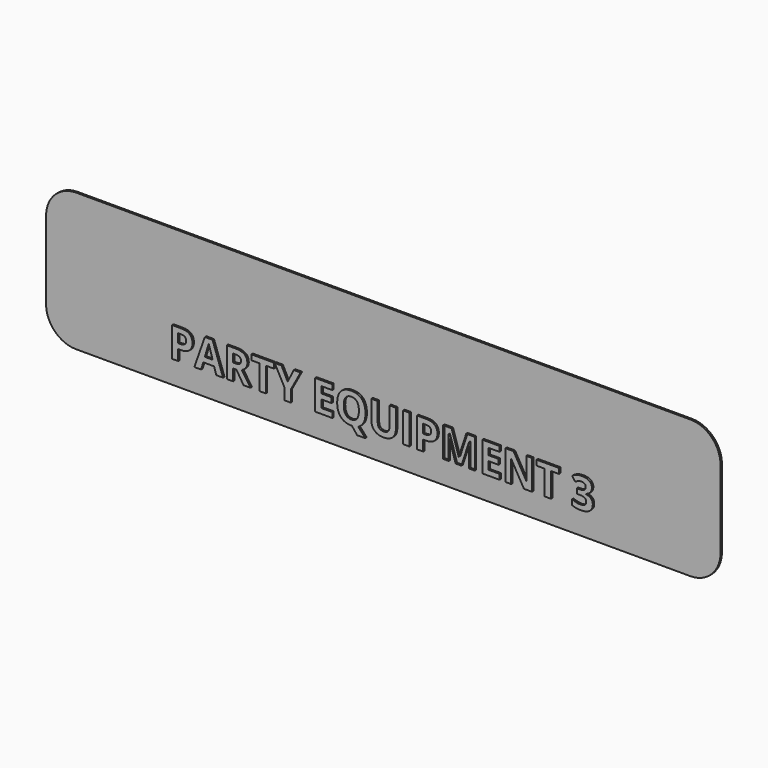
from build123d import *

# Parameters (mm, degrees)
F1_DEPTH     = 0.6
F2_TEXT_SIZE = 13.8888888889
F3_DEPTH     = 0.6


# Not quite as in the source:
# - Text() gives the source's letters only with a copy of the font that has no kerning and outlines rounded to 1/6400 em; it was checked with that copy


with BuildPart() as f1:
    # F0 (on Front) → F1 (new body)
    with BuildSketch(Plane.XZ):
        with BuildLine():
            ThreePointArc((0, 10), (2.9289321881, 2.9289321881), (10, 0))
            Line((10, 0), (215, 0))
            ThreePointArc((215, 0), (222.0710678119, 2.9289321881), (225, 10))
            Line((225, 10), (225, 36))
            ThreePointArc((225, 36), (222.0710678119, 43.0710678119), (215, 46))
            Line((215, 46), (10, 46))
            ThreePointArc((10, 46), (2.9289321881, 43.0710678119), (0, 36))
            Line((0, 36), (0, 10))
        make_face()
    extrude(amount=F1_DEPTH)

    # F2 (on face) → F3 (join)
    with BuildSketch(Plane.XZ.offset(0.6)):
        with Locations((41.2239583333, 8)):
            Text('PARTY EQUIPMENT 3', F2_TEXT_SIZE, font='Open Sans', font_style=FontStyle.BOLD, text_align=(TextAlign.LEFT, TextAlign.BOTTOM))
    extrude(amount=F3_DEPTH)


solid = f1.part
